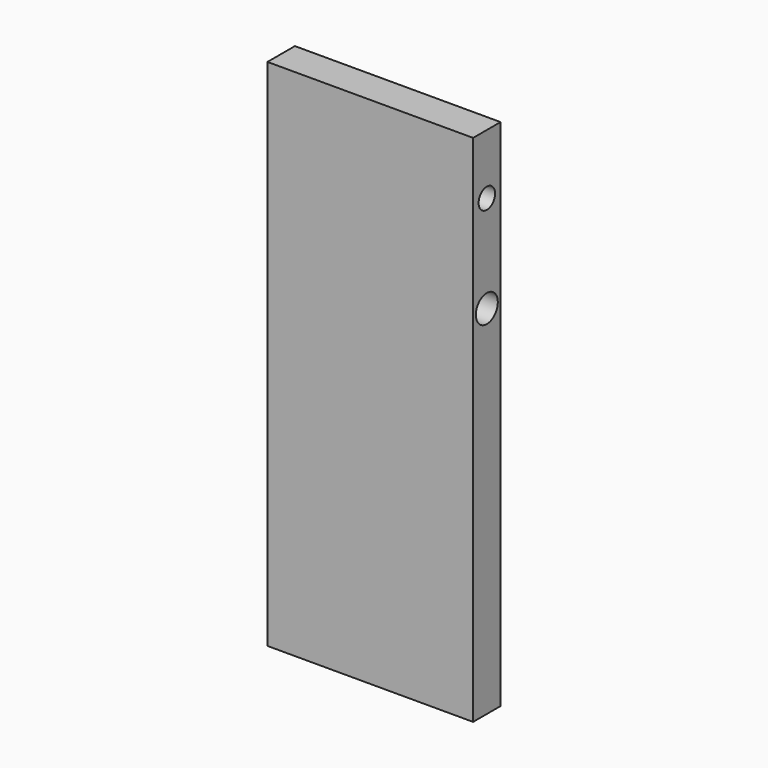
from build123d import *

# Parameters (mm, degrees)
F0_W     = 15.24
F0_H     = 38.1
F1_DEPTH = 1.27
F5_D     = 1.524
F6_R     = 1.016
F7_DEPTH = 15.241


# Not quite as in the source:
# - the program builds the solid bodies; features that only make, move or delete a surface that nothing else refers to are left out


with BuildPart() as f1:
    # F0 (on Front) → F1 (new body, symmetric)
    with BuildSketch(Plane.XZ):
        Rectangle(F0_W, F0_H)
    extrude(amount=F1_DEPTH, both=True)

    # F5 (through all)
    with Locations(Plane.YZ.offset(7.62)):
        with Locations((0, 14.5949712023)):
            Hole(F5_D / 2)

    # F6 (on face) → F7 (cut, through all)
    with BuildSketch(Plane.YZ.offset(7.62)):
        with Locations((0, 7.4023683179)):
            Circle(F6_R)
    extrude(amount=-F7_DEPTH, mode=Mode.SUBTRACT)


solid = f1.part
